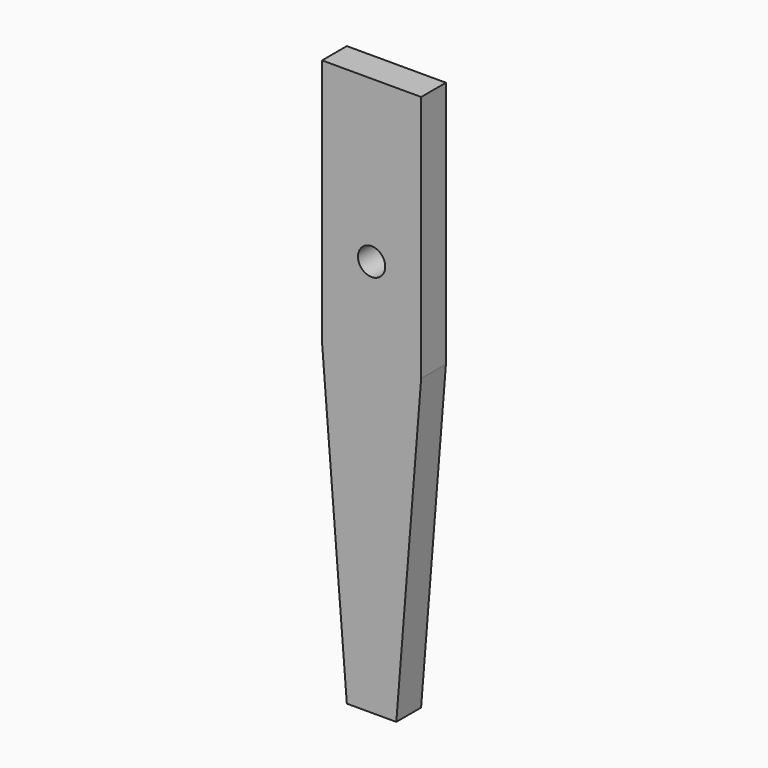
from build123d import *

# Parameters (mm, degrees)
F0_R     = 22
F1_DEPTH = 50


# Not quite as in the source:
# - a feature names something its author has since deleted; it is built from what else it names


with BuildPart() as f1:
    # F0 (on Front) → F1 (new body)
    with BuildSketch(Plane.XZ):
        Polygon((82.7246823907, 255.5227107533), (-77.2753176093, 255.5227107533), (-77.2753176093, -145.831789898), (-37.2753176093, -645.831789898), (42.6163223386, -645.831789898), (82.7246823907, -144.4772892467), align=None)
        with Locations((2.7246823907, -4.4772892467)):
            Circle(F0_R, mode=Mode.SUBTRACT)
    extrude(amount=F1_DEPTH)


solid = f1.part
